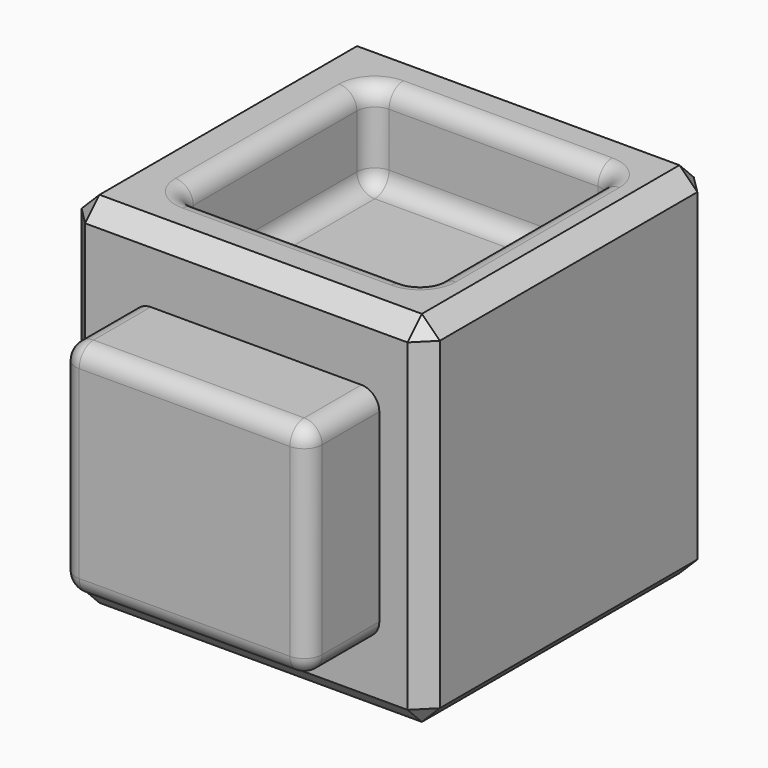
from build123d import *

# Parameters (mm, degrees)
F0_W     = 100.1162827015
F0_H     = 100.4215180874
F1_DEPTH = 100
F2_SIZE  = 5
F3_W     = 68.8809547573
F3_H     = 61.6337545216
F4_DEPTH = 25
F5_R     = 5
F6_W     = 68.3720968664
F6_H     = 67.151170224
F7_DEPTH = 25
F8_R     = 5


with BuildPart() as f1:
    # F0 (on Front) → F1 (new body)
    with BuildSketch(Plane.XZ):
        with Locations((-12.8197669983, -14.4985467196)):
            Rectangle(F0_W, F0_H)
    extrude(amount=F1_DEPTH)

    # F2
    f2_edges = [f1.edges().sort_by_distance(p)[0] for p in [
        (37.238374, -50, -64.709306),
        (-62.877908, -50, 35.712212),
        (-12.819767, -100, 35.712212),
        (-12.819767, 0, 35.712212),
        (37.238374, -50, 35.712212),
        (-12.819767, -100, -64.709306),
        (-12.819767, 0, -64.709306),
        (-62.877908, -100, -14.498547),
        (-62.877908, -50, -64.709306),
        (37.238374, -100, -14.498547),
        (-62.877908, 0, -14.498547),
        (37.238374, 0, -14.498547),
    ]]
    chamfer(f2_edges, length=F2_SIZE)

    # F3 (on face) → F4 (join)
    with BuildSketch(Plane.XZ.offset(100)):
        with Locations((-10.0983185694, -14.7410277277)):
            Rectangle(F3_W, F3_H)
    extrude(amount=F4_DEPTH)

    # F5
    f5_edges = [f1.edges().sort_by_distance(p)[0] for p in [
        (-10.098319, -125, 16.07585),
        (24.342159, -125, -14.741028),
        (24.342159, -112.5, 16.07585),
        (24.342159, -112.5, -45.557905),
        (-10.098319, -125, -45.557905),
        (-44.538796, -112.5, -45.557905),
        (-44.538796, -125, -14.741028),
        (-44.538796, -112.5, 16.07585),
    ]]
    fillet(f5_edges, radius=F5_R)

    # F6 (on face) → F7 (cut)
    with BuildSketch(Plane.XY.offset(35.7122123241)):
        with Locations((-10.5813946575, -50.0290710479)):
            Rectangle(F6_W, F6_H)
    extrude(amount=-F7_DEPTH, mode=Mode.SUBTRACT)

    # F8
    f8_edges = [f1.edges().sort_by_distance(p)[0] for p in [
        (-10.581395, -16.453486, 10.712212),
        (-44.767443, -50.029071, 10.712212),
        (-10.581395, -83.604656, 10.712212),
        (23.604654, -50.029071, 10.712212),
        (23.604654, -16.453486, 23.212212),
        (-44.767443, -16.453486, 23.212212),
        (-44.767443, -83.604656, 23.212212),
        (-44.767443, -50.029071, 35.712212),
        (23.604654, -83.604656, 23.212212),
        (23.604654, -50.029071, 35.712212),
        (-10.581395, -83.604656, 35.712212),
        (-10.581395, -16.453486, 35.712212),
    ]]
    fillet(f8_edges, radius=F8_R)


solid = f1.part
